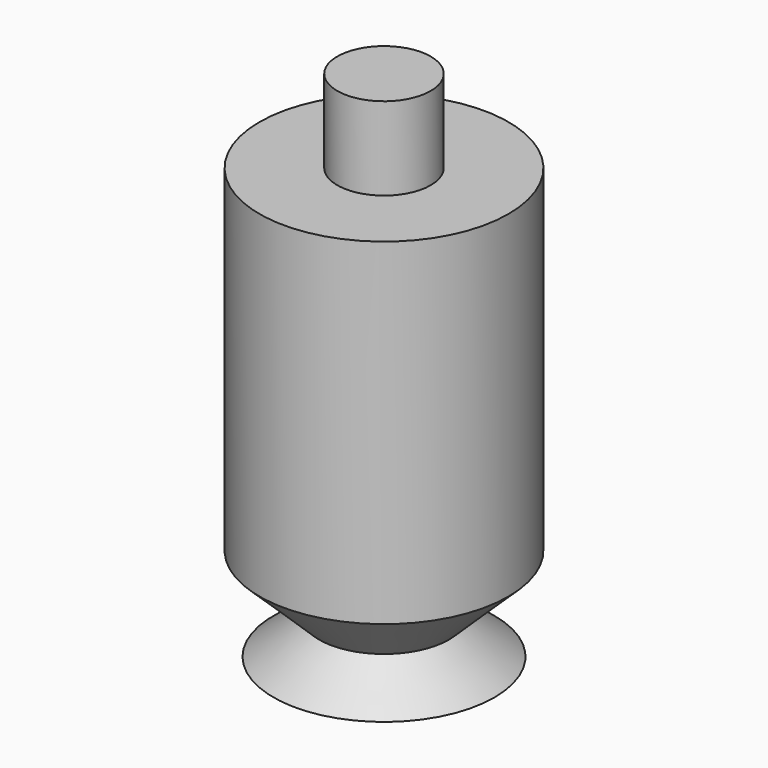
from build123d import *


# Not quite as in the source:
# - a feature names something its author has since deleted; it is built from what else it names


with BuildPart() as f1:
    # F0 (on Front) → F1 (revolve)
    with BuildSketch(Plane.XZ):
        Polygon((3.183866306, 1.7671220925), (6.096, 4.572), (6.096, 21.0566), (2.286, 21.0566), (2.286, 25.1206), (0, 25.1206), (0, 0), (5.4102, 0), align=None)
    revolve(axis=Axis((0, 0, 12.5603), (0, 0, -1)))


solid = f1.part
